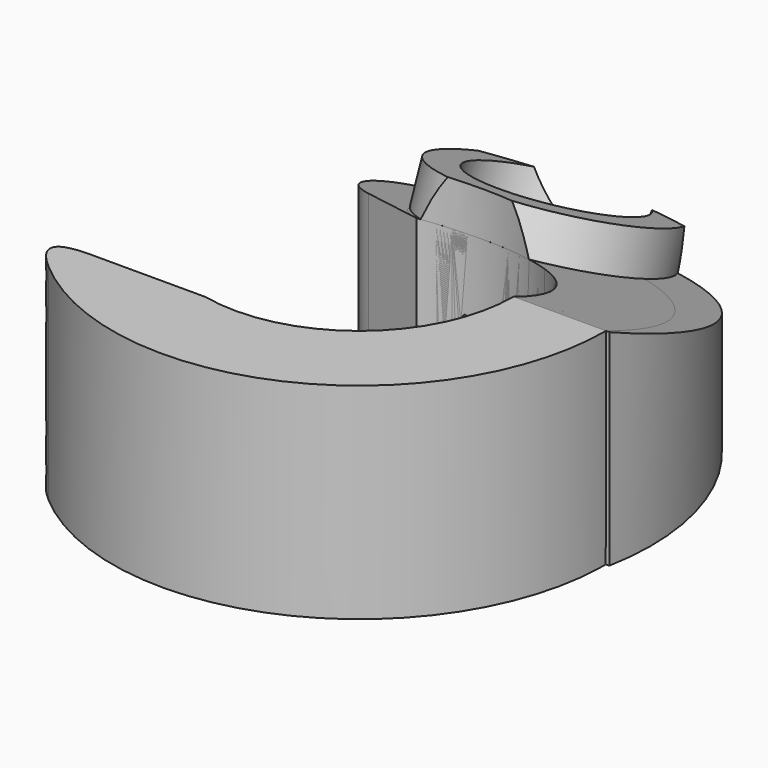
from build123d import *

# Parameters (mm, degrees)
F1_DEPTH       = 10
F2_R           = 24
F2_R_2         = 15
F3_DEPTH       = 10
F5_DEPTH       = 12.5
F6_W           = 22.41528593
F6_H           = 10.1995486766
F7_DEPTH       = 12.5
F12_W          = 51.7317093909
F12_H          = 35.3548980784
F13_DEPTH      = 25
F15_R          = 2.5
F16_DEPTH      = 15
F17_R          = 10.5
F17_R_2        = 7.5
F18_DEPTH      = 4
F19_W          = 61.2675081939
F19_H          = 44.7931201197
F20_DEPTH      = 12.5
F23_T1_DEPTH   = 57.6612211781
F23_2_T1_DEPTH = 77.2316796631
F24_T1_DEPTH   = 44.1608674747
F26_R          = 5.75
F27_DEPTH      = 3.5


# Not quite as in the source:
# - a fillet or chamfer that OpenCascade refuses, or shapes differently, is made with other operations: its cross-section is extruded or revolved along the edge and cut away or added


with BuildPart() as f1:
    # F0 (on Top) → F1 (new body, symmetric)
    with BuildSketch(Plane.XY):
        with BuildLine():
            Line((15, 0), (24.3292674422, 0))
            ThreePointArc((24.3292674422, 0), (0.2560960129, 29.0743140694), (-23.8170754164, 0))
            Line((-23.8170754164, 0), (-15, 0))
            ThreePointArc((-15, 0), (0, 15), (15, 0))
        make_face()
    extrude(amount=F1_DEPTH, both=True)


with BuildPart() as f3:
    # F2 (on Top) → F3 (new body, symmetric)
    with BuildSketch(Plane.XY):
        Circle(F2_R)
        Circle(F2_R_2, mode=Mode.SUBTRACT)
    extrude(amount=F3_DEPTH, both=True)


with BuildPart() as f5:
    # F4 (on Top) → F5 (new body, symmetric)
    with BuildSketch(Plane.XY):
        Polygon((-14.9477146361, -14.5601387329), (-5.1014113761, 13.7780036218), (-24.9381110243, 20.6704159038), (-34.7844142843, -7.6677264509), align=None)
    extrude(amount=F5_DEPTH, both=True)


with BuildPart() as f7:
    # F6 (on Top) → F7 (new body, symmetric)
    with BuildSketch(Plane.XY):
        with Locations((-12.919315137, -9.5406156033)):
            Rectangle(F6_W, F6_H)
    extrude(amount=F7_DEPTH, both=True)


with BuildPart() as f1_1:
    add(f1.part)

    # F8: cut F5, F7
    add(f5.part, mode=Mode.SUBTRACT)
    add(f7.part, mode=Mode.SUBTRACT)


with BuildPart() as f3_1:
    add(f3.part)

    # F8: cut F5, F7
    add(f5.part, mode=Mode.SUBTRACT)
    add(f7.part, mode=Mode.SUBTRACT)


with BuildPart() as f13:
    # F12 (on face) → F13 (new body)
    with BuildSketch(Plane(origin=(0, 3.4732918523, 8.5966990017), x_dir=(1, 0, 0), z_dir=(0, 0.3746065934, 0.9271838546))):
        with Locations((1.7926823348, 13.7932781363)):
            Rectangle(F12_W, F12_H)
    extrude(amount=F13_DEPTH)


with BuildPart() as f3_2:
    add(f3_1.part)

    # F14: cut F13
    add(f13.part, mode=Mode.SUBTRACT)


with BuildPart() as f1_2:
    add(f1_1.part)

    # F14: cut F13
    add(f13.part, mode=Mode.SUBTRACT)


with BuildPart() as f16:
    # F15 (on face) → F16 (new body)
    with BuildSketch(Plane(origin=(0, 3.4732918523, 8.5966990017), x_dir=(1, 0, 0), z_dir=(0, 0.3746065934, 0.9271838546))):
        with Locations((0, 20.4042736441)):
            Circle(F15_R)
    extrude(amount=-F16_DEPTH)


with BuildPart() as f18:
    # F17 (on face) → F18 (new body)
    with BuildSketch(Plane(origin=(0, 3.4732918523, 8.5966990017), x_dir=(1, 0, 0), z_dir=(0, 0.3746065934, 0.9271838546))):
        with Locations((0, 20.4843599349)):
            Circle(F17_R)
        with Locations((0, 20.4843599349)):
            Circle(F17_R_2, mode=Mode.SUBTRACT)
    extrude(amount=F18_DEPTH)


with BuildPart() as f20:
    # F19 (on Top) → F20 (new body, symmetric)
    with BuildSketch(Plane.XY):
        with Locations((-0.9692432359, 18.0722444784)):
            Rectangle(F19_W, F19_H)
        with BuildLine():
            Line((24.173, 0), (15, 0))
            ThreePointArc((15, 0), (0, 15), (-15, 0))
            Line((-15, 0), (-23.85, 0))
            ThreePointArc((-23.85, 0), (0.1615, 29.1552502712), (24.173, 0))
        make_face(mode=Mode.SUBTRACT)
    extrude(amount=F20_DEPTH, both=True)


with BuildPart() as f18_1:
    add(f18.part)

    # F21: cut F20
    add(f20.part, mode=Mode.SUBTRACT)


with BuildPart() as f1_3:
    add(f1_2.part)

    # F22: cut F16
    add(f16.part, mode=Mode.SUBTRACT)

    # F23: fillet of radius 5 on 1 edges, made by hand

    # F23_s2 → F23_t1 (cut)
    with BuildSketch(Plane.XY.offset(-32.6361921936)):
        with BuildLine():
            ThreePointArc((-12.0346234612, 16.1870009336), (-15.3566437884, 20.3034543546), (-13.1237951218, 25.0988057133))
            ThreePointArc((-13.1237951218, 25.0988057133), (-16.6861637402, 22.273317734), (-19.6651630599, 18.8382899979))
            Line((-19.6651630599, 18.8382899979), (-12.0346234612, 16.1870009336))
        make_face()
    extrude(amount=F23_T1_DEPTH, mode=Mode.SUBTRACT)


with BuildPart() as f3_3:
    add(f3_2.part)

    # F22: cut F16
    add(f16.part, mode=Mode.SUBTRACT)

    # F23#2: fillet of radius 5 on 1 edges, made by hand

    # F23_2_s2 → F23_2_t1 (cut)
    with BuildSketch(Plane.XY.offset(-42.1822661383)):
        with BuildLine():
            ThreePointArc((-4.7968588028, 23.5157425064), (-8.7820491741, 19.009568806), (-5.5521549108, 13.9346178938))
            Line((-5.5521549108, 13.9346178938), (-16.2579553104, 17.654429731))
            ThreePointArc((-16.2579553104, 17.654429731), (-10.9277191672, 21.3678486002), (-4.7968588028, 23.5157425064))
        make_face()
    extrude(amount=F23_2_T1_DEPTH, mode=Mode.SUBTRACT)

    # F24: fillet of radius 2 on 1 edges, made by hand

    # F24_s2 → F24_t1 (cut)
    with BuildSketch(Plane.XY.offset(-22.0804337374)):
        with BuildLine():
            add(Edge.make_bspline(
                [(-15.6991416444, -18.1531526636), (-19.7610018026, -14.6403899416), (-14.3908798407, -14.6403899416)],
                knots=[0, 0, 0, 1, 1, 1], degree=2, weights=[1, 1, 1]))
            Line((-14.3908798407, -14.6403899416), (-19.0173337342, -14.6403899416))
            ThreePointArc((-19.0173337342, -14.6403899416), (-17.4468705264, -16.4804947995), (-15.6991416444, -18.1531526636))
        make_face()
    extrude(amount=F24_T1_DEPTH, mode=Mode.SUBTRACT)


with BuildPart() as f27:
    # F26 (on offset) → F27 (new body, symmetric)
    with BuildSketch(Plane(origin=(0, -0.2727740819, -0.675139544), x_dir=(1, 0, 0), z_dir=(0, 0.3746065934, 0.9271838546))):
        with Locations((0, 20.4434879124)):
            Circle(F26_R)
    extrude(amount=F27_DEPTH, both=True)


with BuildPart() as f1_4:
    add(f1_3.part)

    # F28: cut F27
    add(f27.part, mode=Mode.SUBTRACT)


with BuildPart() as f3_4:
    add(f3_3.part)

    # F28: cut F27
    add(f27.part, mode=Mode.SUBTRACT)


solid = Compound([f18_1.part, f1_4.part, f3_4.part])
